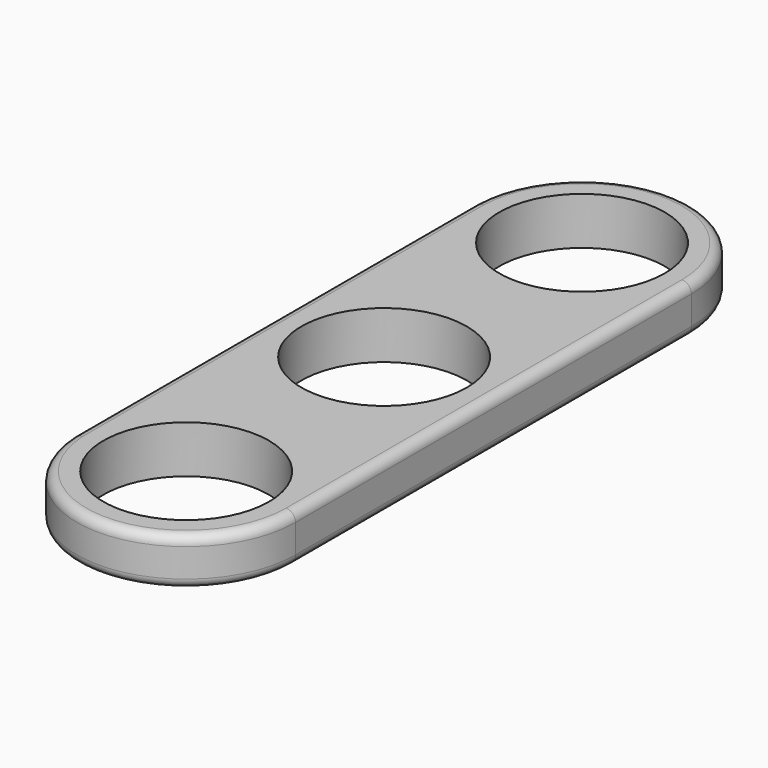
from build123d import *

# Parameters (mm, degrees)
F0_R     = 11.049
F1_DEPTH = 6.35
F2_R     = 1.27


# Not quite as in the source:
# - ends of sketch curves that miss each other by under 0.0002 mm in the source are joined


with BuildPart() as f1:
    # F0 (on Top) → F1 (new body)
    with BuildSketch(Plane.XY):
        with BuildLine():
            ThreePointArc((-14.5963668579, 32.6986430389), (0.1647025721, 18.413606839), (14.6101469387, 33.0177352621))
            ThreePointArc((14.6101469387, 33.0177352621), (0.1647025721, 47.6218636853), (-14.5963668579, 33.3368274853))
            Line((-14.5963668579, 33.3368274853), (-14.5963668579, 32.6986430389))
        make_face()
        with Locations((0.0051469387, 33.0177352621)):
            Circle(F0_R, mode=Mode.SUBTRACT)
        with BuildLine():
            Line((14.59990231, -33.0222639433), (14.6101469387, 33.0177352621))
            ThreePointArc((14.6101469387, 33.0177352621), (0.1647025721, 18.413606839), (-14.5963668579, 32.6986430389))
            Line((-14.5963668579, 32.6986430389), (-14.5963668579, -32.3891018796))
            ThreePointArc((-14.5963668579, -32.3891018796), (0.3115576014, -18.4206970987), (14.59990231, -33.0222639433))
        make_face()
        Circle(F0_R, mode=Mode.SUBTRACT)
        with BuildLine():
            ThreePointArc((14.5999019585, -33.0245295823), (14.5999020903, -33.0233967628), (14.5999021343, -33.0222639432))
            ThreePointArc((14.5999021343, -33.0222639432), (0.3115576014, -18.4206970987), (-14.5963668579, -32.3891018796))
            Line((-14.5963668579, -32.3891018796), (-14.5963668579, -33.6554260069))
            ThreePointArc((-14.5963668579, -33.6554260069), (0.3104250472, -47.6238553049), (14.5999019585, -33.0245295823))
        make_face()
        with Locations((-0.0050978657, -33.0222639432)):
            Circle(F0_R, mode=Mode.SUBTRACT)
    extrude(amount=F1_DEPTH)

    # F2
    f2_edges = [f1.edges().sort_by_distance(p)[0] for p in [
        (14.605025, -0.002264, 0),
        (14.605025, -0.002264, 6.35),
        (0.310425, -47.623855, 0),
        (14.599902, -33.023397, 0),
        (0.164703, 47.621864, 0),
        (0.164703, 47.621864, 6.35),
        (-14.596367, -0.159299, 6.35),
        (0.310425, -47.623855, 6.35),
        (14.599902, -33.023397, 6.35),
        (-14.596367, -0.159299, 0),
    ]]
    fillet(f2_edges, radius=F2_R)


solid = f1.part
